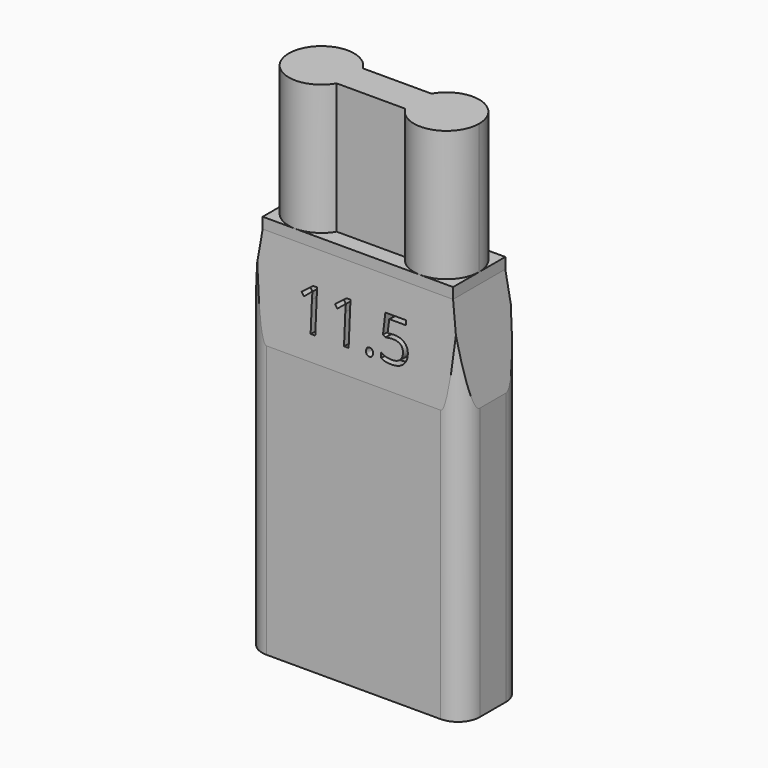
from build123d import *

# Parameters (mm, degrees)
F1_DEPTH     = 12
F4_W         = 20
F4_H         = 7
F5_DEPTH     = 25
F2_W         = 17.5
F2_H         = 6
F6_DEPTH     = 1
F6_FACE_W    = 17.5
F6_FACE_H    = 6
F5_FACE_W    = 20
F5_FACE_H    = 7
F8_TEXT_SIZE = 5.3680909332
F9_DEPTH     = 1
F10_R        = 2


# Not quite as in the source:
# - Text() gives the source's letters only with a copy of the font that has no kerning and outlines rounded to 1/6400 em; it was checked with that copy


with BuildPart() as f1:
    # F0 (on Top) → F1 (new body)
    with BuildSketch(Plane.XY):
        with BuildLine():
            ThreePointArc((-3.1519237886, -1.5), (-2.8522225211, -0.7764571353), (-2.75, 0))
            ThreePointArc((-2.75, 0), (-2.8522225211, 0.7764571353), (-3.1519237886, 1.5))
            Line((-3.1519237886, 1.5), (-3.1519237886, -1.5))
        make_face()
        with BuildLine():
            ThreePointArc((-3.1519237886, 1.5), (-2.8522225211, 0.7764571353), (-2.75, 0))
            ThreePointArc((-2.75, 0), (-2.8522225211, -0.7764571353), (-3.1519237886, -1.5))
            Line((-3.1519237886, -1.5), (3.1519237886, -1.5))
            ThreePointArc((3.1519237886, -1.5), (2.75, 0), (3.1519237886, 1.5))
            Line((3.1519237886, 1.5), (-3.1519237886, 1.5))
        make_face()
        with BuildLine():
            Line((-3.1519237886, -1.5), (-3.1519237886, 1.5))
            ThreePointArc((-3.1519237886, 1.5), (-8.75, 0), (-3.1519237886, -1.5))
        make_face()
        with BuildLine():
            Line((3.1519237886, -1.5), (3.1519237886, 1.5))
            ThreePointArc((3.1519237886, 1.5), (2.75, 0), (3.1519237886, -1.5))
        make_face()
        with BuildLine():
            ThreePointArc((8.75, 0), (6.5264571353, 2.8977774789), (3.1519237886, 1.5))
            Line((3.1519237886, 1.5), (3.1519237886, -1.5))
            ThreePointArc((3.1519237886, -1.5), (6.5264571353, -2.8977774789), (8.75, 0))
        make_face()
    extrude(amount=F1_DEPTH)

    # F2 (on face) → F6 (join)
    with BuildSketch(Plane(origin=(0, 0, 0), x_dir=(1, 0, 0), z_dir=(0, 0, -1))):
        Rectangle(F2_W, F2_H)
    extrude(amount=F6_DEPTH)



with BuildPart() as f5:
    # F4 (on offset) → F5 (new body)
    with BuildSketch(Plane(origin=(0, 0, -10), x_dir=(1, 0, 0), z_dir=(0, 0, -1))):
        Rectangle(F4_W, F4_H)
    extrude(amount=F5_DEPTH)


with BuildPart() as f1_1:
    add(f1.part)

    add(f5.part)  # F7 merges F5
    # F6_face (on face) → F7 section 0
    with BuildSketch(Plane(origin=(0, 0, -1), x_dir=(1, 0, 0), z_dir=(0, 0, -1))):
        Rectangle(F6_FACE_W, F6_FACE_H)
    # F5_face (on face) → F7 section 1
    with BuildSketch(Plane.XY.offset(-10)):
        Rectangle(F5_FACE_W, F5_FACE_H)
    loft()

    # F8 (on face) → F9 (cut)
    with BuildSketch(Plane(origin=(0, -2.9353846154, 0.1630769231), x_dir=(1, 0, 0), z_dir=(0, -0.9984603532, 0.0554700196))):
        with Locations((-5.4922867566, -7.9777319916)):
            Text('11.5', F8_TEXT_SIZE, font='Open Sans', text_align=(TextAlign.LEFT, TextAlign.BOTTOM))
    extrude(amount=-F9_DEPTH, mode=Mode.SUBTRACT)

    # F10
    f10_edges = [f1_1.edges().sort_by_distance(p)[0] for p in [
        (-10, -3.5, -22.5),
        (-10, 3.5, -22.5),
        (10, 3.5, -22.5),
        (10, -3.5, -22.5),
    ]]
    fillet(f10_edges, radius=F10_R)


solid = f1_1.part
